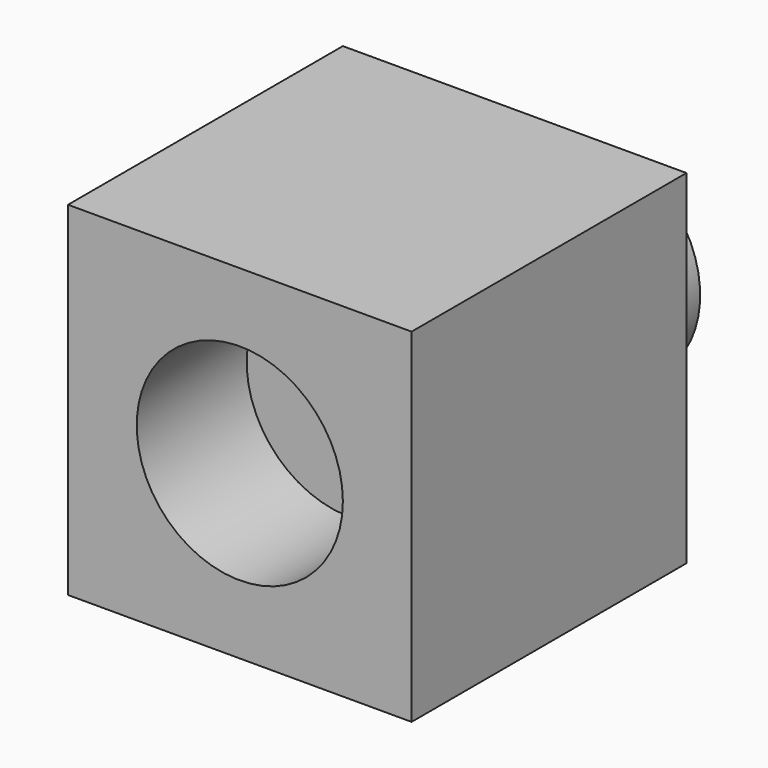
from build123d import *

# Parameters (mm, degrees)
F1_W     = 127
F1_H     = 127
F2_DEPTH = 63.5
F3_R     = 38.1
F4_DEPTH = 50.8
F5_R     = 38.1
F6_DEPTH = 38.1


# Not quite as in the source:
# - a variable given as a bare number and used for a length is read in inches; the dataset says mm whatever the document's units were


with BuildPart() as f2:
    # F1 (on Top) → F2 (new body, symmetric)
    with BuildSketch(Plane.XY):
        Rectangle(F1_W, F1_H)
    extrude(amount=F2_DEPTH, both=True)

    # F3 (on face) → F4 (cut)
    with BuildSketch(Plane.XZ.offset(63.5)):
        Circle(F3_R)
    extrude(amount=-F4_DEPTH, mode=Mode.SUBTRACT)

    # F5 (on face) → F6 (join)
    with BuildSketch(Plane(origin=(0, 63.5, 0), x_dir=(-1, 0, 0), z_dir=(0, 1, 0))):
        Circle(F5_R)
    extrude(amount=F6_DEPTH)


solid = f2.part
